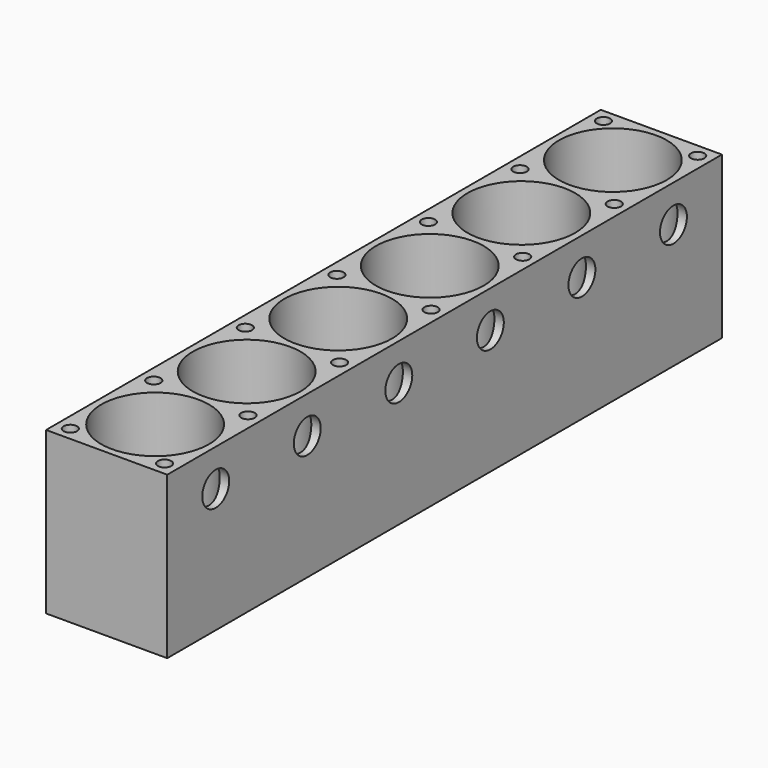
from build123d import *

# Parameters (mm, degrees)
F0_W     = 515
F0_H     = 120
F1_DEPTH = 90
F2_R     = 40
F3_DEPTH = 110
F4_R     = 12.5
F5_DEPTH = 25
F6_R     = 5
F7_DEPTH = 120
F8_DEPTH = 120


# Not quite as in the source:
# - a feature names something its author has since deleted; it is built from what else it names


with BuildPart() as f1:
    # F0 (on Right) → F1 (new body)
    with BuildSketch(Plane.YZ):
        Rectangle(F0_W, F0_H)
    extrude(amount=F1_DEPTH)

    # F2 (on face) → F3 (cut)
    with BuildSketch(Plane.XY.offset(60)):
        with Locations((45, 212.5)):
            Circle(F2_R)
        with Locations((45, 127.5)):
            Circle(F2_R)
        with Locations((45, 42.5)):
            Circle(F2_R)
        with Locations((45, -42.5)):
            Circle(F2_R)
        with Locations((45, -127.5)):
            Circle(F2_R)
        with Locations((45, -212.5)):
            Circle(F2_R)
    extrude(amount=-F3_DEPTH, mode=Mode.SUBTRACT)

    # F4 (on face) → F5 (cut)
    with BuildSketch(Plane.YZ.offset(90)):
        with Locations((-127.5, 32.5)):
            Circle(F4_R)
        with Locations((-212.5, 32.5)):
            Circle(F4_R)
        with Locations((-42.5, 32.5)):
            Circle(F4_R)
        with Locations((42.5, 32.5)):
            Circle(F4_R)
        with Locations((127.5, 32.5)):
            Circle(F4_R)
        with Locations((212.5, 32.5)):
            Circle(F4_R)
    extrude(amount=-F5_DEPTH, mode=Mode.SUBTRACT)

    # F6 (on face) → F7 (cut)
    with BuildSketch(Plane.XY.offset(60)):
        with Locations((80, 170)):
            Circle(F6_R)
        with Locations((80, 247.5)):
            Circle(F6_R)
        with Locations((80, 85)):
            Circle(F6_R)
        with Locations((10, 85)):
            Circle(F6_R)
        with Locations((10, 170)):
            Circle(F6_R)
        with Locations((10, 247.5)):
            Circle(F6_R)
        with Locations((80, 0)):
            Circle(F6_R)
        with Locations((80, -85)):
            Circle(F6_R)
        with Locations((10, -85)):
            Circle(F6_R)
        with Locations((10, -170)):
            Circle(F6_R)
        with Locations((80, -170)):
            Circle(F6_R)
        with Locations((80, -247.5)):
            Circle(F6_R)
        with Locations((10, -247.5)):
            Circle(F6_R)
    extrude(amount=-F7_DEPTH, mode=Mode.SUBTRACT)

    # F6 (on face) → F8 (cut)
    with BuildSketch(Plane.XY.offset(60)):
        with Locations((10, 0)):
            Circle(F6_R)
    extrude(amount=-F8_DEPTH, mode=Mode.SUBTRACT)


solid = f1.part
